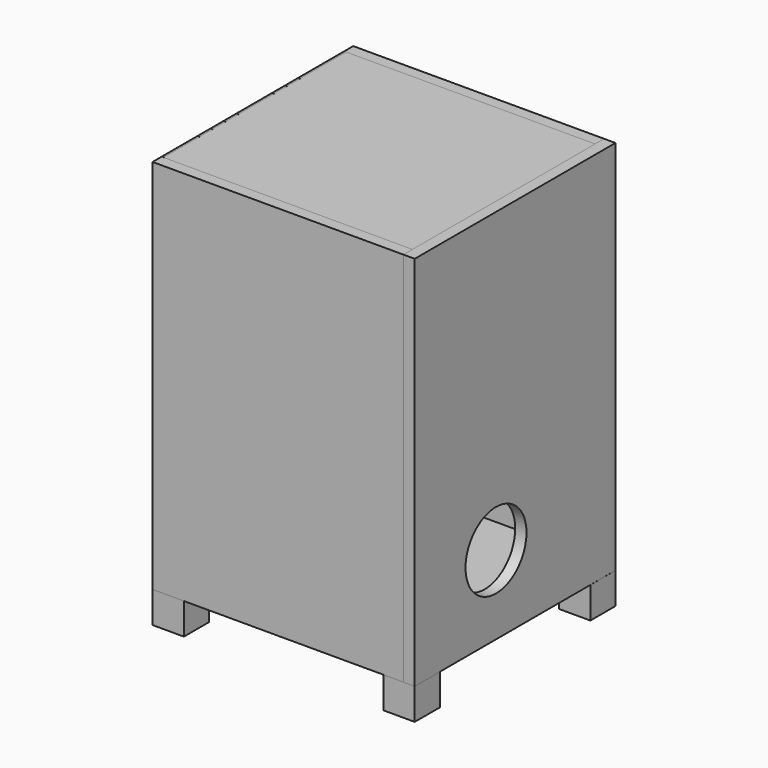
from build123d import *

# Parameters (mm, degrees)
F0_W          = 200
F0_H          = 300
F1_DEPTH      = 9
F2_W          = 1.5
F2_H          = 300
F3_DEPTH      = 191
F5_DEPTH      = 12
F7_DEPTH      = 182
F9_DEPTH      = 12
F10_W         = 20.7938767331
F10_H         = 36.9565486908
F11_DEPTH     = 5
F12_W         = 200
F12_H         = 9
F13_DEPTH     = 182
F14_W         = 200
F14_H         = 9
F15_DEPTH     = 182
F16_W         = 201.5093582915
F16_H         = 300
F17_DEPTH     = 9
F18_W         = 200.0000145435
F18_H         = 300
F19_DEPTH     = 9
F20_R         = 30.3926463741
F21_DEPTH     = 30
F22_W         = 25
F22_H         = 25
F23_DEPTH     = 25
F24_W         = 25
F24_H         = 25
F25_DEPTH     = 25
F26_W         = 25
F26_H         = 25
F27_DEPTH     = 25
F28_W         = 25
F28_H         = 25
F29_DEPTH     = 25
F30_TEXT_SIZE = 32.1829345755
F31_DEPTH     = 1.5


# Not quite as in the source:
# - Text() gives the source's letters only with a copy of the font that has no kerning and outlines rounded to 1/6400 em; it was checked with that copy


with BuildPart() as f1:
    # F0 (on Front) → F1 (new body)
    with BuildSketch(Plane.XZ):
        with Locations((100, 150)):
            Rectangle(F0_W, F0_H)
    extrude(amount=F1_DEPTH)


with BuildPart() as f3:
    # F2 (on Front) → F3 (new body)
    with BuildSketch(Plane.XZ):
        with Locations((0.75, 150)):
            Rectangle(F2_W, F2_H)
    extrude(amount=-F3_DEPTH)


with BuildPart() as f5:
    # F4 (on face) → F5 (new body)
    with BuildSketch(Plane.XZ):
        Polygon((40.8490944999, 104.552505459), (1.5186637909, 129.732005459), (1.5186637909, 79.373005459), align=None)
    extrude(amount=-F5_DEPTH)


with BuildPart() as f7:
    # F6 (on face) → F7 (new body)
    with BuildSketch(Plane.XZ):
        Polygon((1.526577631, 129.7358125448), (40.8490944999, 104.552505459), (45.8840047887, 111.1423218442), (6.8150795943, 136.5261444641), align=None)
    extrude(amount=-F7_DEPTH)


with BuildPart() as f9:
    # F8 (on face) → F9 (new body)
    with BuildSketch(Plane(origin=(0, 182, 0), x_dir=(-1, 0, 0), z_dir=(0, 1, 0))):
        Polygon((-1.526577631, 129.7358125448), (-40.8490944999, 104.552505459), (-1.6243578866, 79.3515220284), align=None)
    extrude(amount=-F9_DEPTH)


with BuildPart() as f11:
    # F10 (on face) → F11 (new body)
    with BuildSketch(Plane(origin=(64.3965065158, 0, 99.1143979187), x_dir=(0.8385512743, 0, -0.5448226871), z_dir=(0.5448226871, 0, 0.8385512743))):
        with Locations((-32.4737061135, 79.5973390341)):
            Rectangle(F10_W, F10_H)
    extrude(amount=F11_DEPTH)


with BuildPart() as f13:
    # F12 (on face) → F13 (new body)
    with BuildSketch(Plane.XZ):
        with Locations((101.5093582915, 295.5)):
            Rectangle(F12_W, F12_H)
    extrude(amount=-F13_DEPTH)


with BuildPart() as f15:
    # F14 (on face) → F15 (new body)
    with BuildSketch(Plane.XZ):
        with Locations((100.0189868084, 4.5)):
            Rectangle(F14_W, F14_H)
    extrude(amount=-F15_DEPTH)


with BuildPart() as f17:
    # F16 (on face) → F17 (new body)
    with BuildSketch(Plane(origin=(0, 182, 0), x_dir=(-1, 0, 0), z_dir=(0, 1, 0))):
        with Locations((-100.7546791458, 150)):
            Rectangle(F16_W, F16_H)
    extrude(amount=F17_DEPTH)


with BuildPart() as f19:
    # F18 (on face) → F19 (new body)
    with BuildSketch(Plane.YZ.offset(200)):
        with Locations((91.0000072718, 150)):
            Rectangle(F18_W, F18_H)
    extrude(amount=F19_DEPTH)

    # F20 (on face) → F21 (cut)
    with BuildSketch(Plane.YZ.offset(209)):
        with Locations((71.9772651792, 62.5780001283)):
            Circle(F20_R)
    extrude(amount=-F21_DEPTH, mode=Mode.SUBTRACT)


with BuildPart() as f23:
    # F22 (on face) → F23 (new body)
    with BuildSketch(Plane(origin=(0, 0, 0), x_dir=(1, 0, 0), z_dir=(0, 0, -1))):
        with Locations((196.5, -3.5)):
            Rectangle(F22_W, F22_H)
    extrude(amount=F23_DEPTH)


with BuildPart() as f25:
    # F24 (on face) → F25 (new body)
    with BuildSketch(Plane(origin=(0, 0, 0), x_dir=(1, 0, 0), z_dir=(0, 0, -1))):
        with Locations((196.5226508603, -178.5)):
            Rectangle(F24_W, F24_H)
    extrude(amount=F25_DEPTH)


with BuildPart() as f27:
    # F26 (on face) → F27 (new body)
    with BuildSketch(Plane(origin=(0, 0, 0), x_dir=(1, 0, 0), z_dir=(0, 0, -1))):
        with Locations((12.5, -3.5)):
            Rectangle(F26_W, F26_H)
    extrude(amount=F27_DEPTH)


with BuildPart() as f29:
    # F28 (on face) → F29 (new body)
    with BuildSketch(Plane(origin=(0, 0, 0), x_dir=(1, 0, 0), z_dir=(0, 0, -1))):
        with Locations((12.5, -178.5)):
            Rectangle(F28_W, F28_H)
    extrude(amount=F29_DEPTH)


with BuildPart() as f31:
    # F30 (on face) → F31 (new body)
    with BuildSketch(Plane(origin=(0, 0, 0), x_dir=(0, -1, 0), z_dir=(-1, 0, 0))):
        with Locations((-190, 165.4216301999)):
            Text('Orange Pear', F30_TEXT_SIZE, font='Open Sans', text_align=(TextAlign.LEFT, TextAlign.BOTTOM))
    extrude(amount=F31_DEPTH)


solid = Compound([f1.part, f3.part, f5.part, f7.part, f9.part, f11.part, f13.part, f15.part, f17.part, f19.part, f23.part, f25.part, f27.part, f29.part, f31.part])
